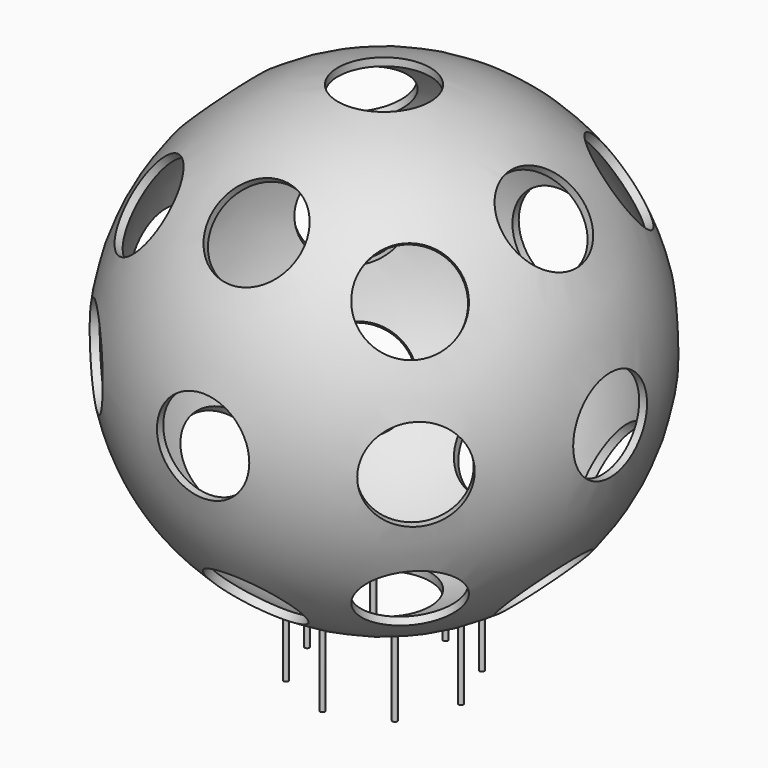
from build123d import *

# Parameters (mm, degrees)
F22_R            = 7.62
F23_DEPTH        = 38.1
F25_R            = 7.62
F26_DEPTH        = 38.1
F26_COPIES_COUNT = 6
F26_COPIES_ANGLE = 225
F28_R            = 7.62
F29_DEPTH        = 38.1
F54_R            = 7.62
F55_DEPTH        = 63.5
F55_COPIES_COUNT = 4
F73_R            = 7.62
F74_DEPTH        = 38.101
F76_R            = 0.4064
F77_DEPTH        = 12.954
F77_COPIES_COUNT = 8


# Not quite as in the source:
# - a feature of the source that left no trace in its solid (it failed there, or was rolled back) is left out
# - a pattern or mirror of a feature is missing from the dataset's text; its kind, count and spacing are read off the source's solid


with BuildPart() as f2:
    # F1 (on Top) → F2 (revolve)
    with BuildSketch(Plane.XY):
        with BuildLine():
            Line((0, -38.1), (0, 38.1))
            ThreePointArc((0, 38.1), (-38.1, 0), (0, -38.1))
        make_face()
    revolve(axis=Axis((0, 0, 0), (0, -1, 0)))

    # F22 (on plane+point) → F23 (cut, symmetric)
    with BuildSketch(Plane.XY.offset(38.1)):
        Circle(F22_R)
    extrude(amount=F23_DEPTH, both=True, mode=Mode.SUBTRACT)

    # F25 (on plane+point) → F26 (cut, symmetric)
    with BuildSketch(Plane.YZ.offset(38.1)):
        Circle(F25_R)
    f26 = extrude(amount=F26_DEPTH, both=True, mode=Mode.SUBTRACT)

    # F26_copies: F26 ×6 about axis
    f26_copies_axis = Axis((0, 0, 0), (0, 0, -1))
    for i in range(1, F26_COPIES_COUNT):
        add(f26.rotate(f26_copies_axis, i * F26_COPIES_ANGLE / (F26_COPIES_COUNT - 1)), mode=Mode.SUBTRACT)

    # F26_copies1: F26 across plane
    add(f26.mirror(Plane(origin=(0, 0, 0), x_dir=(0.9238795325, 0.3826834324, 0), z_dir=(-0.3826834324, 0.9238795325, 0))), mode=Mode.SUBTRACT)

    # F28 (on plane+point) → F29 (cut, symmetric)
    with BuildSketch(Plane.XZ.offset(-38.1)):
        Circle(F28_R)
    extrude(amount=F29_DEPTH, both=True, mode=Mode.SUBTRACT)

    # F42 (on Top) → F43 (revolve, cut)
    with BuildSketch(Plane.XY):
        with BuildLine():
            Line((0, -36.83), (0, 36.83))
            ThreePointArc((0, 36.83), (-36.83, 0), (0, -36.83))
        make_face()
    revolve(axis=Axis((0, 19.05, 0), (0, 1, 0)), mode=Mode.SUBTRACT)

    # F54 (on face) → F55 (cut, symmetric)
    with BuildSketch(Plane(origin=(7.3323484187, -7.3323484187, 7.3323484187), x_dir=(-0.8164965809, -0.4082482905, 0.4082482905), z_dir=(-0.5773502692, 0.5773502692, -0.5773502692))):
        Circle(F54_R)
    f55 = extrude(amount=F55_DEPTH, both=True, mode=Mode.SUBTRACT)

    # F55_copies: F55 ×4 about axis
    f55_copies_axis = Axis((0, 0, 0), (0, 0, 1))
    for i in range(1, F55_COPIES_COUNT):
        add(f55.rotate(f55_copies_axis, i * 360 / F55_COPIES_COUNT), mode=Mode.SUBTRACT)

    # F55_copies1: F55 across plane
    add(f55.mirror(Plane(origin=(0, 0, 0), x_dir=(0, -0.9120955865, -0.4099776106), z_dir=(0.0917517095, 0.4082482905, -0.9082482905))), mode=Mode.SUBTRACT)

    # F55_copies2: F55 across plane
    add(f55.mirror(Plane(origin=(0, 0, 0), x_dir=(0.9756630355, -0.2192752634, 0), z_dir=(0.2141864953, 0.9530206139, 0.2141864953))), mode=Mode.SUBTRACT)

    # F55_copies3: F55 across plane
    add(f55.mirror(Plane(origin=(0, 0, 0), x_dir=(-0.9117817457, 0, 0.4106751127), z_dir=(-0.4088667442, -0.09374123, -0.9077668022))), mode=Mode.SUBTRACT)

    # F55_copies4: F55 across plane
    add(f55.mirror(Plane(origin=(0, 0, 0), x_dir=(-0.2234726459, 0, -0.9747102013), z_dir=(-0.9530060831, -0.2098539363, 0.218496524))), mode=Mode.SUBTRACT)

    # F73 (on Top) → F74 (cut, through all)
    with BuildSketch(Plane.XY):
        Circle(F73_R)
    extrude(amount=-F74_DEPTH, mode=Mode.SUBTRACT)

    # F76 (on offset) → F77 (join)
    with BuildSketch(Plane.XY.offset(-35.56)):
        with Locations((0, -12.7)):
            Circle(F76_R)
    f77 = extrude(amount=-F77_DEPTH)

    # F77_copies: F77 ×8 about axis
    f77_copies_axis = Axis((0, 0, 0), (0, 0, 1))
    for i in range(1, F77_COPIES_COUNT):
        add(f77.rotate(f77_copies_axis, i * 360 / F77_COPIES_COUNT))


solid = f2.part
